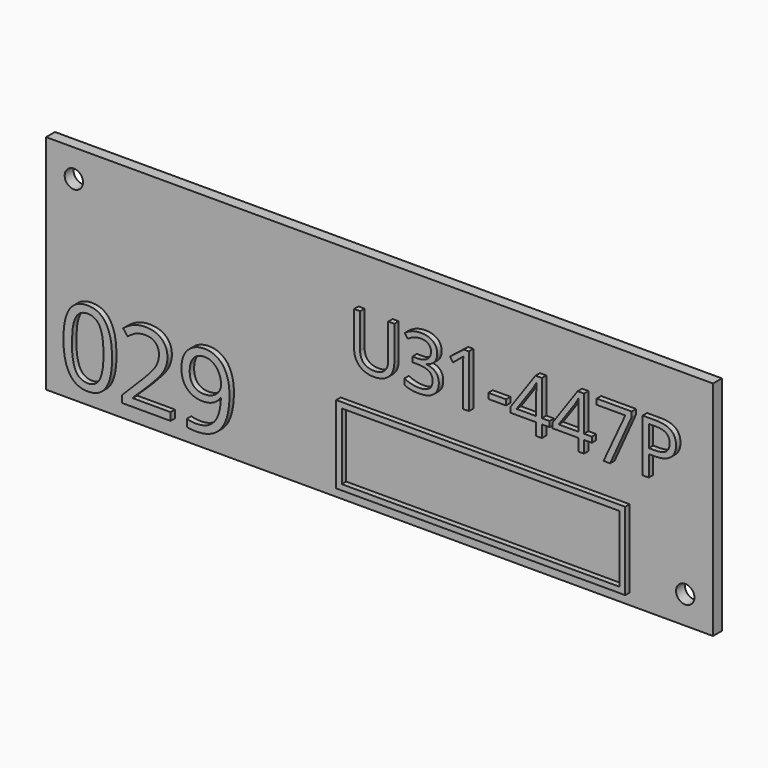
from build123d import *

# Parameters (mm, degrees)
F0_W         = 120
F0_H         = 40
F1_DEPTH     = 2
F3_D         = 3.3
F4_TEXT_SIZE = 13.2628743135
F5_DEPTH     = 1
F6_TEXT_SIZE = 18.5356140827
F7_DEPTH     = 1
F8_W         = 52
F8_H         = 14
F8_W_2       = 49.99999962
F8_H_2       = 11.99999962
F9_DEPTH     = 1


# Not quite as in the source:
# - Text() gives the source's letters only with a copy of the font that has no kerning and outlines rounded to 1/6400 em; it was checked with that copy


with BuildPart() as f1:
    # F0 (on Front) → F1 (new body)
    with BuildSketch(Plane.XZ):
        Rectangle(F0_W, F0_H)
    extrude(amount=F1_DEPTH)

    # F3 (through all)
    with Locations(Plane.XZ.offset(2)):
        with Locations((-55, 15), (55, -15)):
            Hole(F3_D / 2)

    # F4 (on face) → F5 (join)
    with BuildSketch(Plane.XZ.offset(2)):
        with Locations((-5, 2)):
            Text('U31-447P', F4_TEXT_SIZE, font='Open Sans', text_align=(TextAlign.LEFT, TextAlign.BOTTOM))
    extrude(amount=F5_DEPTH)

    # F6 (on face) → F7 (join)
    with BuildSketch(Plane.XZ.offset(2)):
        with Locations((-57, -17)):
            Text('029', F6_TEXT_SIZE, font='Open Sans', text_align=(TextAlign.LEFT, TextAlign.BOTTOM))
    extrude(amount=F7_DEPTH)

    # F8 (on face) → F9 (join)
    with BuildSketch(Plane.XZ.offset(2)):
        with Locations((19, -11)):
            Rectangle(F8_W, F8_H)
        with Locations((19, -11)):
            Rectangle(F8_W_2, F8_H_2, mode=Mode.SUBTRACT)
    extrude(amount=F9_DEPTH)


solid = f1.part
